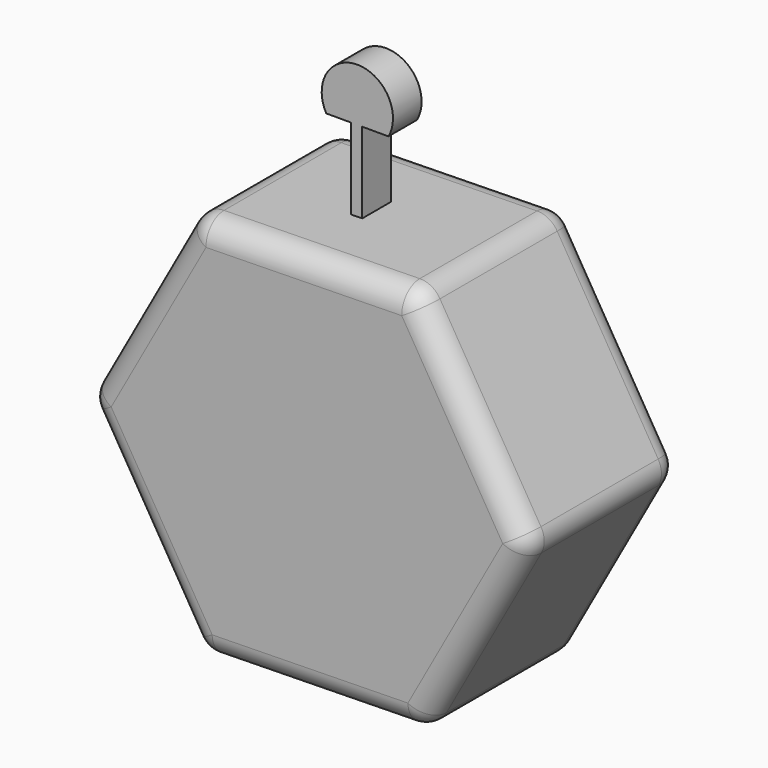
from build123d import *

# Parameters (mm, degrees)
F1_DEPTH = 42.418
F3_START = 17.526
F3_DEPTH = 7.874
F4_F1_R  = 5.08
F4_F2_R  = 5.08
F4_F3_R  = 5.08
F4_F4_R  = 5.08
F4_F5_R  = 5.08
F4_F6_R  = 5.08
F4_F7_R  = 5.08
F4_F8_R  = 5.08


# Not quite as in the source:
# - a feature of the source that left no trace in its solid (it failed there, or was rolled back) is left out


with BuildPart() as f1:
    # F0 (on Front) → F1 (new body)
    with BuildSketch(Plane.XZ):
        Polygon((5.7973779566, -73.3064366429), (29.5106887989, -30.4560707957), (4.2578388349, 11.5054417251), (-44.7083219714, 10.6165883988), (-68.4216328137, -32.2337774485), (-43.1687828497, -74.1952899693), align=None)
    extrude(amount=F1_DEPTH)

    # F2 (on Front) → F3 (join)
    with BuildSketch(Plane.XZ.offset(F3_START)):
        Polygon((-23.4186239541, 28.8229137659), (-23.4186239541, 23.4186165035), (-23.4186239541, -51.1606782675), (-20.8966191858, -54.4032603502), (-20.8966191858, 28.8229137659), align=None)
        with BuildLine():
            Line((-28.8229212165, 28.8229137659), (-23.4186239541, 28.8229137659))
            Line((-23.4186239541, 28.8229137659), (-20.8966191858, 28.8229137659))
            Line((-20.8966191858, 28.8229137659), (-15.1320351288, 28.8229137659))
            ThreePointArc((-15.1320351288, 28.8229137659), (-21.9774781726, 40.5074513695), (-28.8229212165, 28.8229137659))
        make_face()
    extrude(amount=F3_DEPTH)

    # F4: fillet of radius 5.08 on 14 edges, made by hand

    # F4_f1
    f4_f1_edges = [f1.edges().sort_by_distance(p)[0] for p in [
        (5.7973779566, -21.209, -73.3064366429),
    ]]
    fillet(f4_f1_edges, radius=F4_F1_R)

    # F4_f2
    f4_f2_edges = [f1.edges().sort_by_distance(p)[0] for p in [
        (29.5106887989, -21.209, -30.4560707957),
    ]]
    fillet(f4_f2_edges, radius=F4_F2_R)

    # F4_f3
    f4_f3_edges = [f1.edges().sort_by_distance(p)[0] for p in [
        (-43.1687828497, -21.209, -74.1952899693),
    ]]
    fillet(f4_f3_edges, radius=F4_F3_R)

    # F4_f4
    f4_f4_edges = [f1.edges().sort_by_distance(p)[0] for p in [
        (4.2578388349, -21.209, 11.5054417251),
    ]]
    fillet(f4_f4_edges, radius=F4_F4_R)

    # F4_f5
    f4_f5_edges = [f1.edges().sort_by_distance(p)[0] for p in [
        (-68.4216328137, -21.209, -32.2337774485),
    ]]
    fillet(f4_f5_edges, radius=F4_F5_R)

    # F4_f6
    f4_f6_edges = [f1.edges().sort_by_distance(p)[0] for p in [
        (-44.7083219714, -21.209, 10.6165883988),
    ]]
    fillet(f4_f6_edges, radius=F4_F6_R)

    # F4_f7
    f4_f7_edges = [f1.edges().sort_by_distance(p)[0] for p in [
        (-55.7952078317, 0, -53.2145337089),
    ]]
    fillet(f4_f7_edges, radius=F4_F7_R)

    # F4_f8
    f4_f8_edges = [f1.edges().sort_by_distance(p)[0] for p in [
        (-55.7952078317, -42.418, -53.2145337089),
    ]]
    fillet(f4_f8_edges, radius=F4_F8_R)


solid = f1.part
